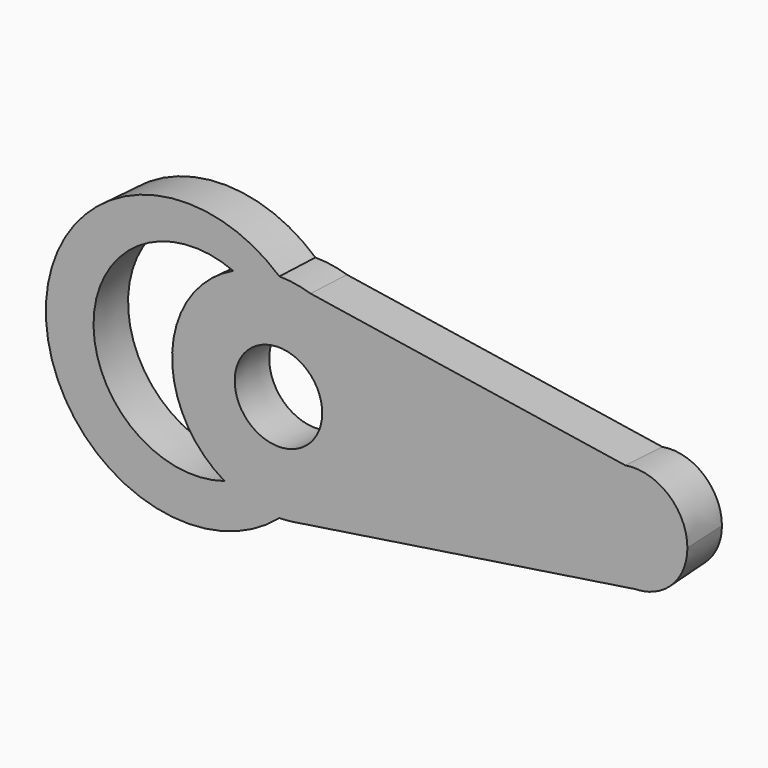
from build123d import *

# Parameters (mm, degrees)
F0_R                   = 25.4
F1_DEPTH               = 25.4
DRAFT_F1_DRAFTED_ANGLE = -3
F2_DEPTH               = 25.4
F3_DEPTH               = 25.4


# Not quite as in the source:
# - an extrude with a draft is written as a straight extrude whose walls are then drafted


with BuildPart() as f1:
    # F0 (on Front) → F1 (new body)
    with BuildSketch(Plane.XZ):
        with BuildLine():
            Line((17.339507874, 54.4560737355), (0, 57.15))
            ThreePointArc((0, 57.15), (-11.0230653317, 56.0768627037), (-21.6321582215, 52.8977526052))
            ThreePointArc((-21.6321582215, 52.8977526052), (-57.088837484, 2.643318884), (-26.4276524327, -50.672494382))
            ThreePointArc((-26.4276524327, -50.672494382), (-13.6049521511, -55.5070065574), (0, -57.15))
            ThreePointArc((0, -57.15), (5.2215891174, -56.9109612209), (10.3994980148, -56.1958445175))
            ThreePointArc((10.3994980148, -56.1958445175), (43.9343476767, -36.5499055297), (57.15, 0))
            ThreePointArc((57.15, 0), (46.136077938, 33.7281012288), (17.339507874, 54.4560737355))
        make_face()
        Circle(F0_R, mode=Mode.SUBTRACT)
        with BuildLine():
            ThreePointArc((17.339507874, 54.4560737355), (8.7737644719, 56.4725026627), (0, 57.15))
            Line((0, 57.15), (17.339507874, 54.4560737355))
        make_face()
        with BuildLine():
            ThreePointArc((-21.6321582215, 52.8977526052), (-11.0230653317, 56.0768627037), (0, 57.15))
            ThreePointArc((0, 57.15), (-126.6015624758, 0), (0, -57.15))
            ThreePointArc((0, -57.15), (-13.6049521511, -55.5070065574), (-26.4276524327, -50.672494382))
            ThreePointArc((-26.4276524327, -50.672494382), (-102.9784222642, 4.7680916307), (-21.6321582215, 52.8977526052))
        make_face()
        with BuildLine():
            Line((190.7515645497, 27.5141733394), (17.339507874, 54.4560737355))
            ThreePointArc((17.339507874, 54.4560737355), (46.136077938, 33.7281012288), (57.15, 0))
            ThreePointArc((57.15, 0), (43.9343476767, -36.5499055297), (10.3994980148, -56.1958445175))
            Line((10.3994980148, -56.1958445175), (196.2111575178, -27.9335529497))
            ThreePointArc((196.2111575178, -27.9335529497), (167.8054383757, -2.7378383186), (190.7515645497, 27.5141733394))
        make_face()
        with BuildLine():
            ThreePointArc((223.5509745393, 0), (213.5674731524, 21.4057879452), (190.7515645497, 27.5141733394))
            ThreePointArc((190.7515645497, 27.5141733394), (167.8054383757, -2.7378383186), (196.2111575178, -27.9335529497))
            Line((196.2111575178, -27.9335529497), (203.3432786767, -26.8487443417))
            ThreePointArc((203.3432786767, -26.8487443417), (217.9345515107, -16.8018305908), (223.5509745393, 0))
        make_face()
        with BuildLine():
            Line((203.3432786767, -26.8487443417), (196.2111575178, -27.9335529497))
            ThreePointArc((196.2111575178, -27.9335529497), (199.812377616, -27.6223064241), (203.3432786767, -26.8487443417))
        make_face()
    extrude(amount=F1_DEPTH)

    # draft_F1_drafted
    draft_f1_drafted_walls = [f1.faces().sort_by_distance(p)[0] for p in [
        (-57.088837484, -16.9333333333, 2.643318884),
        (-102.9784222642, -16.9333333333, 4.7680916307),
        (5.2215891174, -16.9333333333, -56.9109612209),
        (103.3053277663, -16.9333333333, -42.0646987336),
        (223.4165107028, -16.9333333333, 2.7378383186),
        (104.0455362118, -16.9333333333, 40.9851235375),
        (8.7737644719, -16.9333333333, 56.4725026627),
        (-126.6015624758, -16.9333333333, 0),
        (-25.4, -16.9333333333, 0),
    ]]
    draft(draft_f1_drafted_walls, neutral_plane=Plane.XZ, angle=DRAFT_F1_DRAFTED_ANGLE)

    # F0 (on Front) → F2 (join)
    with BuildSketch(Plane.XZ):
        with BuildLine():
            Line((17.339507874, 54.4560737355), (0, 57.15))
            ThreePointArc((0, 57.15), (-11.0230653317, 56.0768627037), (-21.6321582215, 52.8977526052))
            ThreePointArc((-21.6321582215, 52.8977526052), (-57.088837484, 2.643318884), (-26.4276524327, -50.672494382))
            ThreePointArc((-26.4276524327, -50.672494382), (-13.6049521511, -55.5070065574), (0, -57.15))
            ThreePointArc((0, -57.15), (5.2215891174, -56.9109612209), (10.3994980148, -56.1958445175))
            ThreePointArc((10.3994980148, -56.1958445175), (43.9343476767, -36.5499055297), (57.15, 0))
            ThreePointArc((57.15, 0), (46.136077938, 33.7281012288), (17.339507874, 54.4560737355))
        make_face()
        Circle(F0_R, mode=Mode.SUBTRACT)
        with BuildLine():
            ThreePointArc((17.339507874, 54.4560737355), (8.7737644719, 56.4725026627), (0, 57.15))
            Line((0, 57.15), (17.339507874, 54.4560737355))
        make_face()
        with BuildLine():
            ThreePointArc((-21.6321582215, 52.8977526052), (-11.0230653317, 56.0768627037), (0, 57.15))
            ThreePointArc((0, 57.15), (-126.6015624758, 0), (0, -57.15))
            ThreePointArc((0, -57.15), (-13.6049521511, -55.5070065574), (-26.4276524327, -50.672494382))
            ThreePointArc((-26.4276524327, -50.672494382), (-102.9784222642, 4.7680916307), (-21.6321582215, 52.8977526052))
        make_face()
        with BuildLine():
            Line((190.7515645497, 27.5141733394), (17.339507874, 54.4560737355))
            ThreePointArc((17.339507874, 54.4560737355), (46.136077938, 33.7281012288), (57.15, 0))
            ThreePointArc((57.15, 0), (43.9343476767, -36.5499055297), (10.3994980148, -56.1958445175))
            Line((10.3994980148, -56.1958445175), (196.2111575178, -27.9335529497))
            ThreePointArc((196.2111575178, -27.9335529497), (167.8054383757, -2.7378383186), (190.7515645497, 27.5141733394))
        make_face()
        with BuildLine():
            ThreePointArc((223.5509745393, 0), (213.5674731524, 21.4057879452), (190.7515645497, 27.5141733394))
            ThreePointArc((190.7515645497, 27.5141733394), (167.8054383757, -2.7378383186), (196.2111575178, -27.9335529497))
            Line((196.2111575178, -27.9335529497), (203.3432786767, -26.8487443417))
            ThreePointArc((203.3432786767, -26.8487443417), (217.9345515107, -16.8018305908), (223.5509745393, 0))
        make_face()
        with BuildLine():
            Line((203.3432786767, -26.8487443417), (196.2111575178, -27.9335529497))
            ThreePointArc((196.2111575178, -27.9335529497), (199.812377616, -27.6223064241), (203.3432786767, -26.8487443417))
        make_face()
    extrude(amount=F2_DEPTH)

    # F0 (on Front) → F3 (join)
    with BuildSketch(Plane.XZ):
        with BuildLine():
            Line((17.339507874, 54.4560737355), (0, 57.15))
            ThreePointArc((0, 57.15), (-11.0230653317, 56.0768627037), (-21.6321582215, 52.8977526052))
            ThreePointArc((-21.6321582215, 52.8977526052), (-57.088837484, 2.643318884), (-26.4276524327, -50.672494382))
            ThreePointArc((-26.4276524327, -50.672494382), (-13.6049521511, -55.5070065574), (0, -57.15))
            ThreePointArc((0, -57.15), (5.2215891174, -56.9109612209), (10.3994980148, -56.1958445175))
            ThreePointArc((10.3994980148, -56.1958445175), (43.9343476767, -36.5499055297), (57.15, 0))
            ThreePointArc((57.15, 0), (46.136077938, 33.7281012288), (17.339507874, 54.4560737355))
        make_face()
        Circle(F0_R, mode=Mode.SUBTRACT)
        with BuildLine():
            ThreePointArc((17.339507874, 54.4560737355), (8.7737644719, 56.4725026627), (0, 57.15))
            Line((0, 57.15), (17.339507874, 54.4560737355))
        make_face()
        with BuildLine():
            ThreePointArc((-21.6321582215, 52.8977526052), (-11.0230653317, 56.0768627037), (0, 57.15))
            ThreePointArc((0, 57.15), (-126.6015624758, 0), (0, -57.15))
            ThreePointArc((0, -57.15), (-13.6049521511, -55.5070065574), (-26.4276524327, -50.672494382))
            ThreePointArc((-26.4276524327, -50.672494382), (-102.9784222642, 4.7680916307), (-21.6321582215, 52.8977526052))
        make_face()
        with BuildLine():
            Line((190.7515645497, 27.5141733394), (17.339507874, 54.4560737355))
            ThreePointArc((17.339507874, 54.4560737355), (46.136077938, 33.7281012288), (57.15, 0))
            ThreePointArc((57.15, 0), (43.9343476767, -36.5499055297), (10.3994980148, -56.1958445175))
            Line((10.3994980148, -56.1958445175), (196.2111575178, -27.9335529497))
            ThreePointArc((196.2111575178, -27.9335529497), (167.8054383757, -2.7378383186), (190.7515645497, 27.5141733394))
        make_face()
        with BuildLine():
            ThreePointArc((223.5509745393, 0), (213.5674731524, 21.4057879452), (190.7515645497, 27.5141733394))
            ThreePointArc((190.7515645497, 27.5141733394), (167.8054383757, -2.7378383186), (196.2111575178, -27.9335529497))
            Line((196.2111575178, -27.9335529497), (203.3432786767, -26.8487443417))
            ThreePointArc((203.3432786767, -26.8487443417), (217.9345515107, -16.8018305908), (223.5509745393, 0))
        make_face()
        with BuildLine():
            Line((203.3432786767, -26.8487443417), (196.2111575178, -27.9335529497))
            ThreePointArc((196.2111575178, -27.9335529497), (199.812377616, -27.6223064241), (203.3432786767, -26.8487443417))
        make_face()
    extrude(amount=F3_DEPTH)


solid = f1.part
